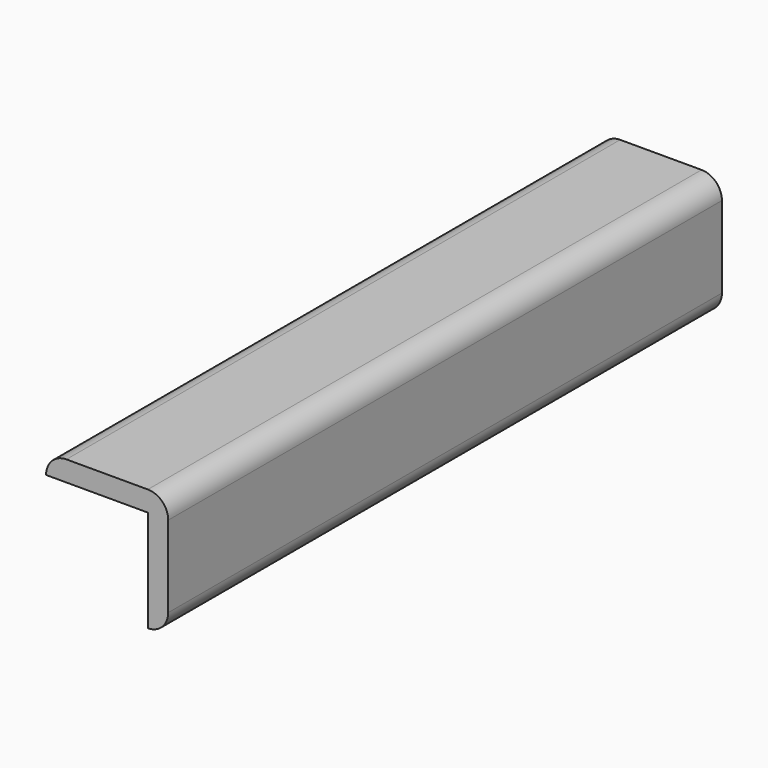
from build123d import *

# Parameters (mm, degrees)
F1_DEPTH = 85
F2_R     = 4.99999


# Not quite as in the source:
# - a fillet or chamfer is up to 0.001 mm smaller than in the source, because OpenCascade refuses the exact size


with BuildPart() as f1:
    # F0 (on Front) → F1 (new body, symmetric)
    with BuildSketch(Plane.XZ):
        Polygon((15, 15), (-15, 15), (-15, 10), (10, 10), (10, -15), (15, -15), align=None)
    extrude(amount=F1_DEPTH, both=True)

    # F2 (radius 5 in the source; OpenCascade refuses exactly that, so slightly less here)
    f2_edges = [f1.edges().sort_by_distance(p)[0] for p in [
        (-15, 0, 15),
        (15, 0, 15),
        (15, 0, -15),
    ]]
    fillet(f2_edges, radius=F2_R)


solid = f1.part
